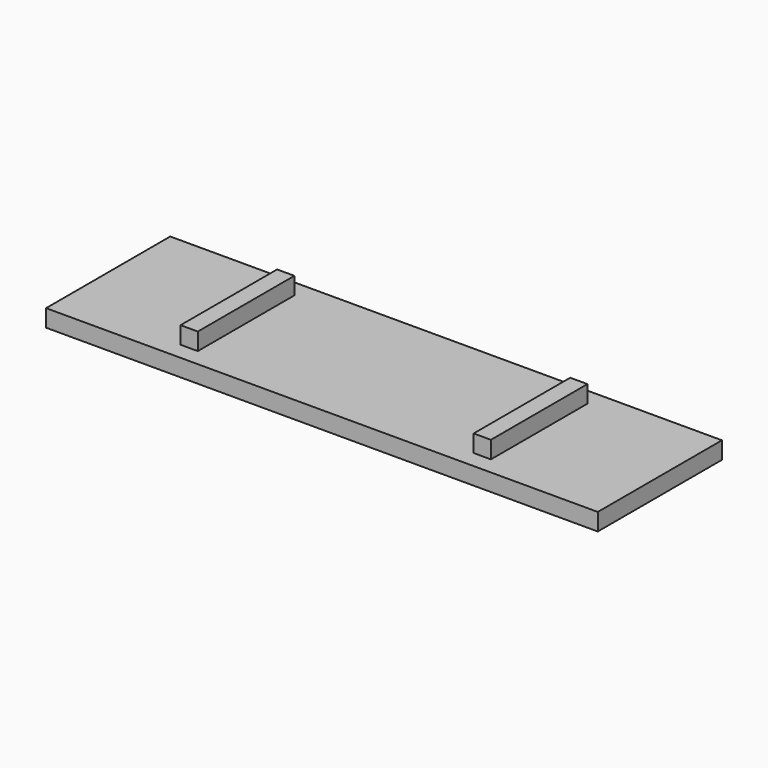
from build123d import *

# Parameters (mm, degrees)
F0_W     = 1
F0_H     = 1
F1_DEPTH = 9
F2_W     = 1
F2_H     = 1
F3_DEPTH = 1
F4_W     = 1
F4_H     = 1
F5_DEPTH = 1


with BuildPart() as f1:
    # F0 (on Front) → F1 (new body)
    with BuildSketch(Plane.XZ):
        Polygon((-9, 1), (-16, 1), (-16, 0), (16, 0), (16, 1), (9, 1), (8, 1), (-8, 1), align=None)
        with Locations((-8.5, 1.5)):
            Rectangle(F0_W, F0_H)
        with Locations((8.5, 1.5)):
            Rectangle(F0_W, F0_H)
    extrude(amount=F1_DEPTH)

    # F2 (on face) → F3 (cut)
    with BuildSketch(Plane.XZ.offset(9)):
        Polygon((-9.9123697728, 3.1492931303), (-9.9123697728, 1), (-9, 1), (-9, 2), (-8, 2), (-8, 1), (8, 1), (8, 2), (9, 2), (9, 1), (10.0291045383, 1), (10.0291045383, 3.1492931303), align=None)
        with Locations((-8.5, 1.5)):
            Rectangle(F2_W, F2_H)
        with Locations((8.5, 1.5)):
            Rectangle(F2_W, F2_H)
    extrude(amount=-F3_DEPTH, mode=Mode.SUBTRACT)

    # F4 (on face) → F5 (cut)
    with BuildSketch(Plane(origin=(0, 0, 0), x_dir=(-1, 0, 0), z_dir=(0, 1, 0))):
        with Locations((-8.5, 1.5)):
            Rectangle(F4_W, F4_H)
        with Locations((8.5, 1.5)):
            Rectangle(F4_W, F4_H)
    extrude(amount=-F5_DEPTH, mode=Mode.SUBTRACT)


solid = f1.part
